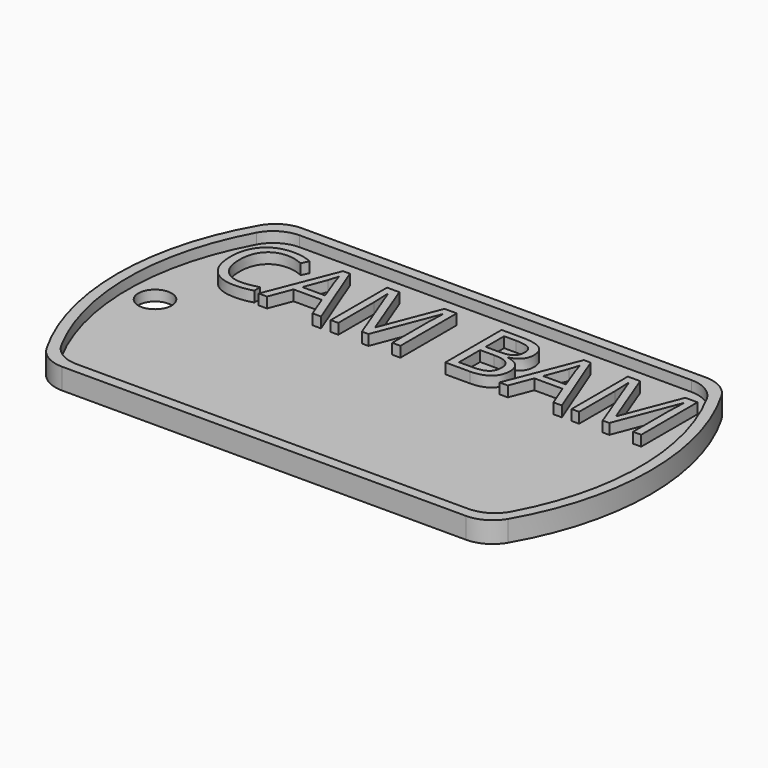
from build123d import *

# Parameters (mm, degrees)
F1_DEPTH     = 1
F3_DEPTH     = 1
F4_R         = 1.5875
F5_DEPTH     = 1
F6_TEXT_SIZE = 9.3908453386
F7_DEPTH     = 1


# Not quite as in the source:
# - Text() gives the source's letters only with a copy of the font that has no kerning and outlines rounded to 1/6400 em; it was checked with that copy


with BuildPart() as f1:
    # F0 (on Top) → F1 (new body)
    with BuildSketch(Plane.XY):
        with BuildLine():
            ThreePointArc((-19.2474145991, 14.2875), (-20.8349145991, 13.862130657), (-21.9970452561, 12.7))
            ThreePointArc((-21.9970452561, 12.7), (-25.4, 0), (-21.9970452561, -12.7))
            ThreePointArc((-21.9970452561, -12.7), (-20.8349145991, -13.862130657), (-19.2474145991, -14.2875))
            Line((-19.2474145991, -14.2875), (19.2474145991, -14.2875))
            ThreePointArc((19.2474145991, -14.2875), (20.8349145991, -13.862130657), (21.9970452561, -12.7))
            ThreePointArc((21.9970452561, -12.7), (25.4, 0), (21.9970452561, 12.7))
            ThreePointArc((21.9970452561, 12.7), (20.8349145991, 13.862130657), (19.2474145991, 14.2875))
            Line((19.2474145991, 14.2875), (-19.2474145991, 14.2875))
        make_face()
    extrude(amount=F1_DEPTH)

    # F2 (on face) → F3 (join)
    with BuildSketch(Plane.XY.offset(1)):
        with BuildLine():
            Line((19.2474145991, 14.2875), (-19.2474145991, 14.2875))
            ThreePointArc((-19.2474145991, 14.2875), (-20.8349145991, 13.862130657), (-21.9970452561, 12.7))
            ThreePointArc((-21.9970452561, 12.7), (-25.4, 0), (-21.9970452561, -12.7))
            ThreePointArc((-21.9970452561, -12.7), (-20.8349145991, -13.862130657), (-19.2474145991, -14.2875))
            Line((-19.2474145991, -14.2875), (19.2474145991, -14.2875))
            ThreePointArc((19.2474145991, -14.2875), (20.8349145991, -13.862130657), (21.9970452561, -12.7))
            ThreePointArc((21.9970452561, -12.7), (25.4, 0), (21.9970452561, 12.7))
            ThreePointArc((21.9970452561, 12.7), (20.8349145991, 13.862130657), (19.2474145991, 14.2875))
        make_face()
        with BuildLine():
            ThreePointArc((-21.4526124879, 11.6252061249), (-20.2856017842, 12.8404540819), (-18.6611352482, 13.2875))
            Line((-18.6611352482, 13.2875), (18.6611352482, 13.2875))
            ThreePointArc((18.6611352482, 13.2875), (20.2856017842, 12.8404540819), (21.4526124879, 11.6252061249))
            ThreePointArc((21.4526124879, 11.6252061249), (24.4, 0), (21.4526124879, -11.6252061249))
            ThreePointArc((21.4526124879, -11.6252061249), (20.2856017842, -12.8404540819), (18.6611352482, -13.2875))
            Line((18.6611352482, -13.2875), (-18.6611352482, -13.2875))
            ThreePointArc((-18.6611352482, -13.2875), (-20.2856017842, -12.8404540819), (-21.4526124879, -11.6252061249))
            ThreePointArc((-21.4526124879, -11.6252061249), (-24.4, 0), (-21.4526124879, 11.6252061249))
        make_face(mode=Mode.SUBTRACT)
    extrude(amount=F3_DEPTH)

    # F4 (on face) → F5 (cut)
    with BuildSketch(Plane.XY.offset(1)):
        with Locations((-21.821282804, 0)):
            Circle(F4_R)
    extrude(amount=-F5_DEPTH, mode=Mode.SUBTRACT)

    # F6 (on face) → F7 (join)
    with BuildSketch(Plane.XY.offset(1)):
        with Locations((-21.1180629694, 4.0670571266)):
            Text('CAM BAM', F6_TEXT_SIZE, font='Open Sans', text_align=(TextAlign.LEFT, TextAlign.BOTTOM))
    extrude(amount=F7_DEPTH)


solid = f1.part
